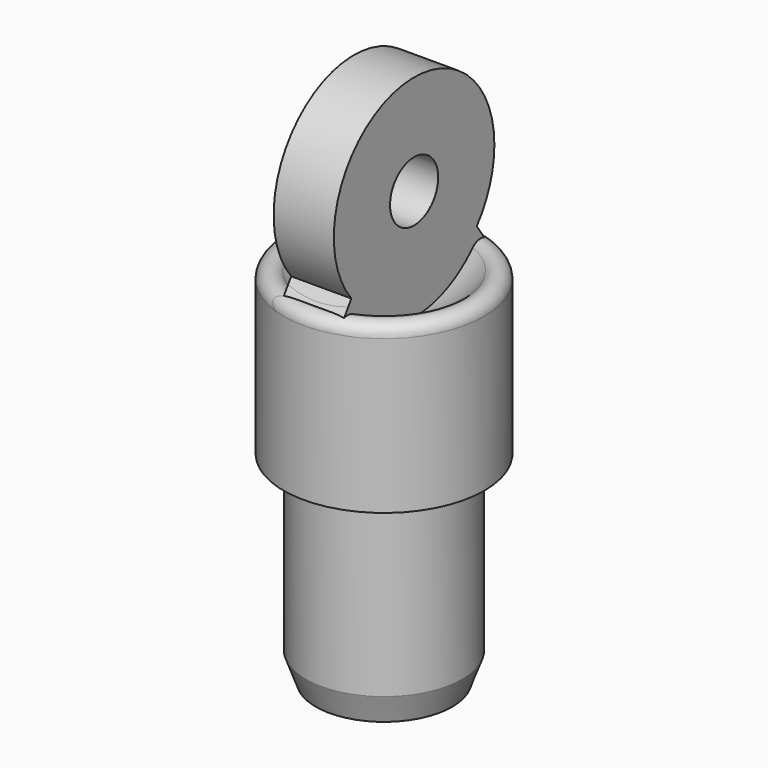
from build123d import *

# Parameters (mm, degrees)
F0_R         = 12.7
F1_DEPTH     = 25.4
F4_R         = 3.81
F5_DEPTH     = 3.81
F6_T4_ANGLE  = 90
F6_T9_ANGLE  = 90
F6_T14_ANGLE = 270
F6_T19_ANGLE = 270
F6_T24_ANGLE = 270
F6_T29_ANGLE = 270
F7_R         = 9.906
F8_DEPTH     = 25.4
F9_SIZE2     = 3.4892963227
F9_SIZE      = 1.27


# Not quite as in the source:
# - a fillet or chamfer that OpenCascade refuses, or shapes differently, is made with other operations: its cross-section is extruded or revolved along the edge and cut away or added


with BuildPart() as f1:
    # F0 (on Top) → F1 (new body)
    with BuildSketch(Plane.XY):
        Circle(F0_R)
    extrude(amount=F1_DEPTH)

    # F2 (on Right) → F3 (revolve, cut)
    with BuildSketch(Plane.YZ):
        with BuildLine():
            Line((0, 15.875), (0, 42.545))
            ThreePointArc((0, 42.545), (-13.335, 29.21), (0, 15.875))
        make_face()
    revolve(axis=Axis((0, 0, 25.198931613), (0, 0, 1)), mode=Mode.SUBTRACT)

    # F4 (on Right) → F5 (join, symmetric)
    with BuildSketch(Plane.YZ):
        with BuildLine():
            ThreePointArc((9.9246541198, 22.5559075849), (11.9860983502, 26.2819711364), (12.7, 30.48))
            ThreePointArc((12.7, 30.48), (-4.1980288636, 42.4660983502), (-9.9246541198, 22.5559075849))
            ThreePointArc((-9.9246541198, 22.5559075849), (0, 17.78), (9.9246541198, 22.5559075849))
        make_face()
        with Locations((0, 30.48)):
            Circle(F4_R, mode=Mode.SUBTRACT)
        with BuildLine():
            ThreePointArc((9.9246541198, 22.5559075849), (0, 17.78), (-9.9246541198, 22.5559075849))
            Line((-9.9246541198, 22.5559075849), (-12.0323663577, 19.4415319711))
            ThreePointArc((-12.0323663577, 19.4415319711), (-6.795833015, 14.9780300529), (0, 13.9006329783))
            ThreePointArc((0, 13.9006329783), (6.795833015, 14.9780300529), (12.0323663577, 19.4415319711))
            Line((12.0323663577, 19.4415319711), (9.9246541198, 22.5559075849))
        make_face()
    extrude(amount=F5_DEPTH, both=True)

    # F6: fillet of radius 1.524 on 2 edges, made by hand


with BuildPart() as f6_tool2:
    # F6_s3 → F6_t4 (revolve)
    with BuildSketch(Plane.XZ):
        with BuildLine():
            ThreePointArc((12.7, 19.4178140847), (11.7125077962, 20.8442555958), (10.0297435897, 20.4221408452))
            ThreePointArc((10.0297435897, 20.4221408452), (11.6075121114, 22.645863531), (12.7, 25.1440161092))
            Line((12.7, 25.1440161092), (12.7, 19.4178140847))
        make_face()
    revolve(axis=Axis((0, 0, 25.1440161092), (0, 0, -1)), revolution_arc=F6_T4_ANGLE)

    split(bisect_by=Plane.YZ.offset(3.81), keep=Keep.TOP)


with BuildPart() as f1_1:
    add(f1.part)

    # F6_t1: cut F6_tool2
    add(f6_tool2.part, mode=Mode.SUBTRACT)


with BuildPart() as f6_tool7:
    # F6_s8 → F6_t9 (revolve)
    with BuildSketch(Plane.XZ):
        with BuildLine():
            ThreePointArc((12.7, 19.4178140847), (11.7125077962, 20.8442555958), (10.0297435897, 20.4221408452))
            ThreePointArc((10.0297435897, 20.4221408452), (11.6075121114, 22.645863531), (12.7, 25.1440161092))
            Line((12.7, 25.1440161092), (12.7, 19.4178140847))
        make_face()
    revolve(axis=Axis((0, 0, 25.1440161092), (0, 0, -1)), revolution_arc=F6_T9_ANGLE)

    split(bisect_by=Plane(origin=(0, -17.2767572385, 11.6923702143), x_dir=(1, 0, 0), z_dir=(0, -0.8281687795, 0.5604787887)), keep=Keep.TOP)


with BuildPart() as f1_2:
    add(f1_1.part)

    # F6_t6: cut F6_tool7
    add(f6_tool7.part, mode=Mode.SUBTRACT)


with BuildPart() as f6_tool12:
    # F6_s13 → F6_t14 (revolve)
    with BuildSketch(Plane.YZ):
        with BuildLine():
            ThreePointArc((-12.7, 19.4178140847), (-11.7125077962, 20.8442555958), (-10.0297435897, 20.4221408452))
            ThreePointArc((-10.0297435897, 20.4221408452), (-11.6075121114, 22.645863531), (-12.7, 25.1440161092))
            Line((-12.7, 25.1440161092), (-12.7, 19.4178140847))
        make_face()
    revolve(axis=Axis((0, 0, 25.1440161092), (0, 0, -1)), revolution_arc=F6_T14_ANGLE)

    split(bisect_by=Plane(origin=(0, -17.2767572385, 11.6923702143), x_dir=(1, 0, 0), z_dir=(0, -0.8281687795, 0.5604787887)), keep=Keep.TOP)


with BuildPart() as f1_3:
    add(f1_2.part)

    # F6_t11: cut F6_tool12
    add(f6_tool12.part, mode=Mode.SUBTRACT)


with BuildPart() as f6_tool17:
    # F6_s18 → F6_t19 (revolve)
    with BuildSketch(Plane.YZ):
        with BuildLine():
            ThreePointArc((-12.7, 19.4178140847), (-11.7125077962, 20.8442555958), (-10.0297435897, 20.4221408452))
            ThreePointArc((-10.0297435897, 20.4221408452), (-11.6075121114, 22.645863531), (-12.7, 25.1440161092))
            Line((-12.7, 25.1440161092), (-12.7, 19.4178140847))
        make_face()
    revolve(axis=Axis((0, 0, 25.1440161092), (0, 0, -1)), revolution_arc=F6_T19_ANGLE)

    split(bisect_by=Plane.YZ.offset(-3.81), keep=Keep.BOTTOM)


with BuildPart() as f1_4:
    add(f1_3.part)

    # F6_t16: cut F6_tool17
    add(f6_tool17.part, mode=Mode.SUBTRACT)


with BuildPart() as f6_tool22:
    # F6_s23 → F6_t24 (revolve)
    with BuildSketch(Plane.YZ):
        with BuildLine():
            ThreePointArc((-12.7, 19.4178140847), (-11.7125077962, 20.8442555958), (-10.0297435897, 20.4221408452))
            ThreePointArc((-10.0297435897, 20.4221408452), (-11.6075121114, 22.645863531), (-12.7, 25.1440161092))
            Line((-12.7, 25.1440161092), (-12.7, 19.4178140847))
        make_face()
    revolve(axis=Axis((0, 0, 25.1440161092), (0, 0, -1)), revolution_arc=F6_T24_ANGLE)

    split(bisect_by=Plane.YZ.offset(3.81), keep=Keep.TOP)


with BuildPart() as f1_5:
    add(f1_4.part)

    # F6_t21: cut F6_tool22
    add(f6_tool22.part, mode=Mode.SUBTRACT)


with BuildPart() as f6_tool27:
    # F6_s28 → F6_t29 (revolve)
    with BuildSketch(Plane.YZ):
        with BuildLine():
            ThreePointArc((-12.7, 19.4178140847), (-11.7125077962, 20.8442555958), (-10.0297435897, 20.4221408452))
            ThreePointArc((-10.0297435897, 20.4221408452), (-11.6075121114, 22.645863531), (-12.7, 25.1440161092))
            Line((-12.7, 25.1440161092), (-12.7, 19.4178140847))
        make_face()
    revolve(axis=Axis((0, 0, 25.1440161092), (0, 0, -1)), revolution_arc=F6_T29_ANGLE)

    split(bisect_by=Plane(origin=(0, 17.2767572385, 11.6923702143), x_dir=(1, 0, 0), z_dir=(0, 0.8281687795, 0.5604787887)), keep=Keep.TOP)


with BuildPart() as f1_6:
    add(f1_5.part)

    # F6_t26: cut F6_tool27
    add(f6_tool27.part, mode=Mode.SUBTRACT)

    # F7 (on face) → F8 (join)
    with BuildSketch(Plane(origin=(0, 0, 0), x_dir=(1, 0, 0), z_dir=(0, 0, -1))):
        Circle(F7_R)
    extrude(amount=F8_DEPTH)

    # F9
    f9_edges = [f1_6.edges().sort_by_distance(p)[0] for p in [
        (-9.906, 0, -25.4),
    ]]
    f9_side = f1_6.faces().sort_by_distance((0, 0, -25.4))[0]
    chamfer(f9_edges, length=F9_SIZE, length2=F9_SIZE2, reference=f9_side)


solid = f1_6.part
